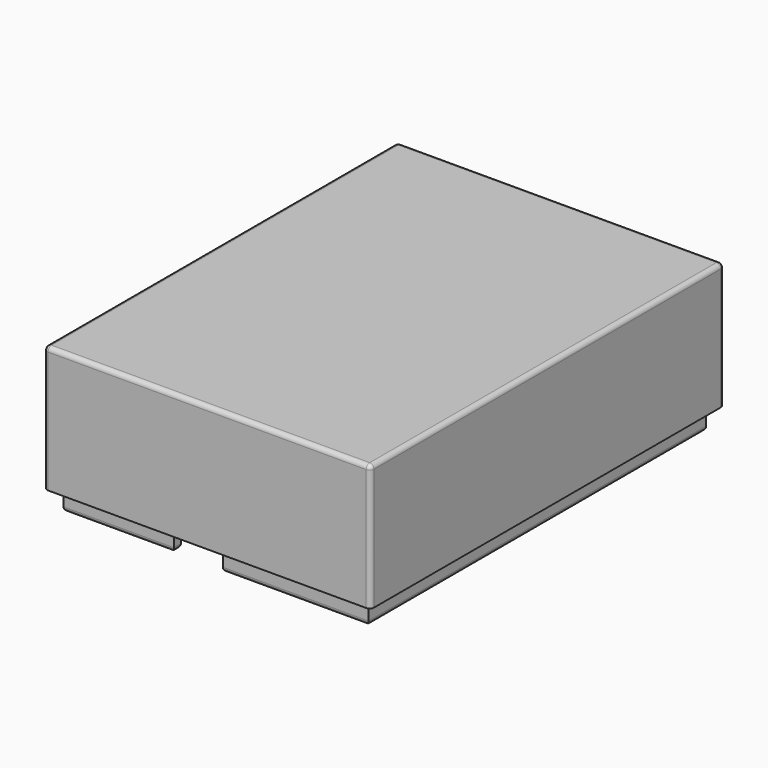
from build123d import *

# Parameters (mm, degrees)
F0_W         = 7
F0_H         = 2.3
F1_DEPTH     = 29
F2_DEPTH     = 5
F4_DEPTH     = 2
F5_R         = 0.99999
F6_TEXT_SIZE = 18.458672437
F7_DEPTH     = 0.5


# Not quite as in the source:
# - a fillet or chamfer is up to 0.001 mm smaller than in the source, because OpenCascade refuses the exact size
# - Text() gives the source's letters only with a copy of the font that has no kerning and outlines rounded to 1/6400 em; it was checked with that copy


with BuildPart() as f1:
    # F0 (on Top) → F1 (new body)
    with BuildSketch(Plane.XY):
        Polygon((-7, 48.5), (-7, 50.8), (-37, 50.8), (-37, -50.8), (-7, -50.8), (-7, -48.1331741877), (-9.3, -48.0424538255), (-34.7, -48.0424538255), (-34.7, 48.5), (-9.3, 48.5), align=None)
        with Locations((-3.5, 49.65)):
            Rectangle(F0_W, F0_H)
        Polygon((38.1, 50.8), (0, 50.8), (0, 48.5), (2.3, 48.5), (35.8, 48.5), (35.8, -48.5), (2.3, -48.5), (0, -48.4092796378), (0, -50.8), (38.1, -50.8), align=None)
        Polygon((0, -50.8), (0, -48.4092796378), (-7, -48.1331741877), (-7, -50.8), align=None)
        Polygon((-9.3, 46.5), (-9.3, 48.5), (-34.7, 48.5), (-34.7, -48.0424538255), (-9.3, -48.0424538255), (-9.3, -46.0424538255), (-32.7, -46.0424538255), (-32.7, 46.5), align=None)
        Polygon((35.8, 48.5), (2.3, 48.5), (2.3, 46.5), (33.8, 46.5), (33.8, -46.5), (2.3, -46.5), (2.3, -48.5), (35.8, -48.5), align=None)
    extrude(amount=F1_DEPTH)

    # F0 (on Top) → F2 (join)
    with BuildSketch(Plane.XY):
        Polygon((-9.3, 46.5), (-9.3, 48.5), (-34.7, 48.5), (-34.7, -48.0424538255), (-9.3, -48.0424538255), (-9.3, -46.0424538255), (-32.7, -46.0424538255), (-32.7, 46.5), align=None)
        Polygon((35.8, 48.5), (2.3, 48.5), (2.3, 46.5), (33.8, 46.5), (33.8, -46.5), (2.3, -46.5), (2.3, -48.5), (35.8, -48.5), align=None)
    extrude(amount=-F2_DEPTH)

    # F3 (on face) → F4 (join)
    with BuildSketch(Plane.XY.offset(29)):
        Polygon((2.3, 48.5), (-9.3, 48.5), (-9.3, 46.5), (-32.7, 46.5), (-32.7, -46.0424538255), (-9.3, -46.0424538255), (-9.3, -48.0424538255), (2.3, -48.5), (2.3, -46.5), (33.8, -46.5), (33.8, 46.5), (2.3, 46.5), align=None)
    extrude(amount=-F4_DEPTH)

    # F5 (radius 1 in the source; OpenCascade refuses exactly that, so slightly less here)
    f5_edges = [f1.edges().sort_by_distance(p)[0] for p in [
        (18.05, 46.5, -5),
        (19.05, 48.5, -5),
        (35.8, 0, -5),
        (33.8, 0, -5),
        (18.05, -46.5, -5),
        (19.05, -48.5, -5),
        (-21, -46.042454, -5),
        (-22, -48.042454, -5),
        (-32.7, 0.228773, -5),
        (-34.7, 0.228773, -5),
        (-21, 46.5, -5),
        (-22, 48.5, -5),
        (-9.3, 47.5, -5),
        (2.3, 47.5, -5),
        (2.3, -47.5, -5),
        (-9.3, -47.042454, -5),
        (0.55, 50.8, 29),
        (38.1, 0, 29),
        (0.55, -50.8, 29),
        (-37, 0, 29),
        (-37, -50.8, 14.5),
        (-37, 50.8, 14.5),
        (38.1, 50.8, 14.5),
        (38.1, -50.8, 14.5),
    ]]
    fillet(f5_edges, radius=F5_R)

    # F6 (on face) → F7 (cut)
    with BuildSketch(Plane(origin=(0, 0, 27), x_dir=(1, 0, 0), z_dir=(0, 0, -1))):
        with Locations((-14.5185170695, -7.0194960572)):
            Text('idk', F6_TEXT_SIZE, font='Open Sans', font_style=FontStyle.BOLD, text_align=(TextAlign.LEFT, TextAlign.BOTTOM))
    extrude(amount=-F7_DEPTH, mode=Mode.SUBTRACT)


solid = f1.part
